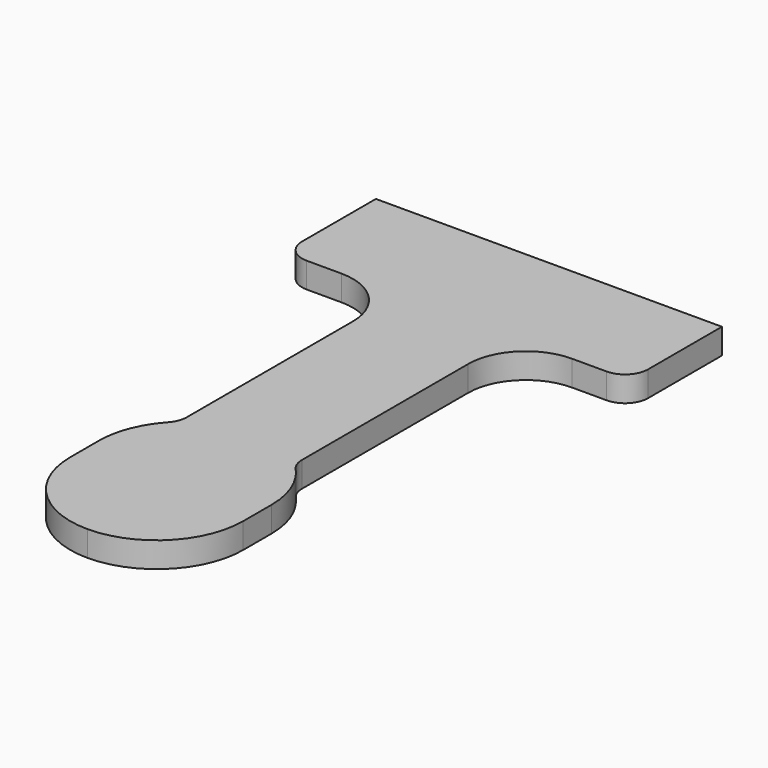
from build123d import *

# Parameters (mm, degrees)
F0_W     = 25.4
F0_H     = 63.5
F1_DEPTH = 5.588
F2_R     = 5.08
F3_R     = 12.7
F4_R     = 5.08
F5_R     = 19.04999


# Not quite as in the source:
# - a fillet or chamfer is up to 0.001 mm smaller than in the source, because OpenCascade refuses the exact size


with BuildPart() as f1:
    # F0 (on Top) → F1 (new body)
    with BuildSketch(Plane.XY):
        Polygon((38.1, 12.7), (-38.1, 12.7), (-38.1, -12.7), (-12.7, -12.7), (12.7, -12.7), (38.1, -12.7), align=None)
        with Locations((0, -44.45)):
            Rectangle(F0_W, F0_H)
        Polygon((12.7, -76.2), (-12.7, -76.2), (-19.05, -76.2), (-19.05, -114.3), (19.05, -114.3), (19.05, -76.2), align=None)
    extrude(amount=F1_DEPTH)

    # F2
    f2_edges = [f1.edges().sort_by_distance(p)[0] for p in [
        (-38.1, -12.7, 2.794),
        (38.1, -12.7, 2.794),
    ]]
    fillet(f2_edges, radius=F2_R)

    # F3
    f3_edges = [f1.edges().sort_by_distance(p)[0] for p in [
        (-12.7, -12.7, 2.794),
        (12.7, -12.7, 2.794),
    ]]
    fillet(f3_edges, radius=F3_R)

    # F4
    f4_edges = [f1.edges().sort_by_distance(p)[0] for p in [
        (-12.7, -76.2, 2.794),
        (12.7, -76.2, 2.794),
    ]]
    fillet(f4_edges, radius=F4_R)

    # F5 (radius 19.05 in the source; OpenCascade refuses exactly that, so slightly less here)
    f5_edges = [f1.edges().sort_by_distance(p)[0] for p in [
        (-19.05, -114.3, 2.794),
        (-19.05, -76.2, 2.794),
        (19.05, -114.3, 2.794),
        (19.05, -76.2, 2.794),
    ]]
    fillet(f5_edges, radius=F5_R)


solid = f1.part
